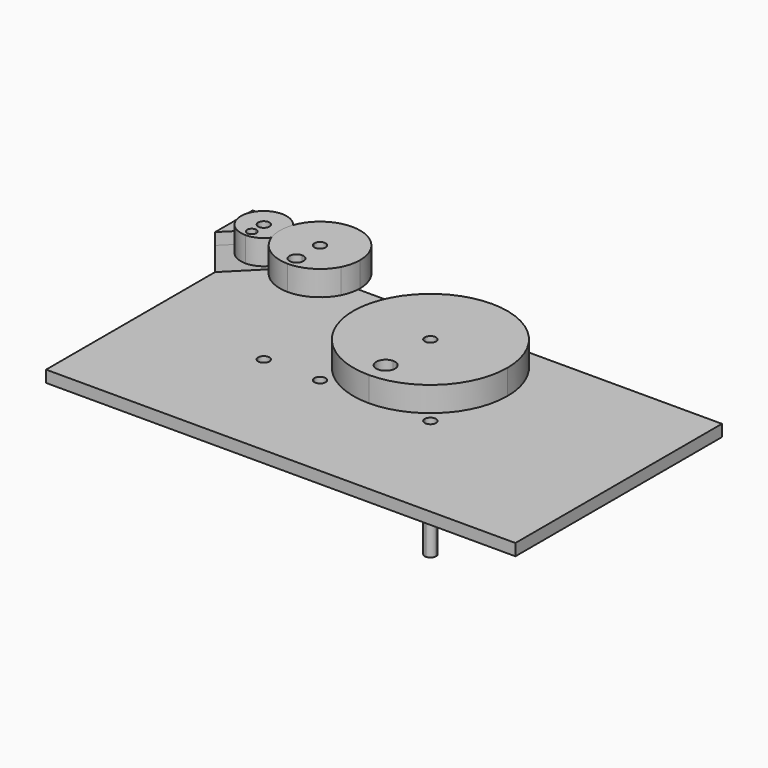
from build123d import *

# Parameters (mm, degrees)
F0_W     = 12.7
F0_H     = 6.35
F1_DEPTH = 3.175
F2_START = 25.4
F2_DEPTH = 6.731
F3_START = 25.4
F3_DEPTH = 6.731
F4_START = 12.7
F4_DEPTH = 6.731
F5_START = -6.35
F5_DEPTH = 25.4
F6_DEPTH = 6.35
F7_DEPTH = 3.175
F8_DEPTH = 6.35
F9_DEPTH = 3.175


# Not quite as in the source:
# - a feature names something its author has since deleted; it is built from what else it names


with BuildPart() as f1:
    # F0 (on Top) → F1 (new body)
    with BuildSketch(Plane.XY):
        Polygon((-53.6384286517, 34.5555226523), (-53.6384286517, 40.9055226523), (-66.3384286517, 28.2055226523), (-66.3384286517, -28.9444773477), (60.6615713483, -28.9444773477), (60.6615713483, 40.9055226523), (-40.9384286517, 40.9055226523), (-40.9384286517, 34.5555226523), align=None)
        with BuildLine():
            ThreePointArc((-33.3374786517, -2.7570773477), (-37.7198436388, -0.9418423348), (-39.5350786517, 3.4405226523))
            ThreePointArc((-39.5350786517, 3.4405226523), (-35.2680968666, 9.3297466308), (-28.3426948036, 7.1096342711))
            ThreePointArc((-28.3426948036, 7.1096342711), (-18.8492977605, 14.2746971722), (-8.4843562027, 8.4411133425))
            ThreePointArc((-8.4843562027, 8.4411133425), (14.2662795753, 24.1284571428), (32.5882213483, 3.4405226523))
            ThreePointArc((32.5882213483, 3.4405226523), (26.484121643, -11.2960776424), (11.7475213483, -17.4001773477))
            ThreePointArc((11.7475213483, -17.4001773477), (-1.1000263962, -12.9690871372), (-8.4843562027, -1.5600680379))
            ThreePointArc((-8.4843562027, -1.5600680379), (-12.5449573003, -5.8757972031), (-18.2667243218, -7.4170245234))
            ThreePointArc((-18.2667243218, -7.4170245234), (-24.4292066664, -5.3990050059), (-28.3426948036, -0.2285889665))
            ThreePointArc((-28.3426948036, -0.2285889665), (-30.5383216722, -2.0889407904), (-33.3374786517, -2.7570773477))
        make_face(mode=Mode.SUBTRACT)
        with BuildLine():
            ThreePointArc((32.5882213483, 3.4405226523), (14.2662795753, 24.1284571428), (-8.4843562027, 8.4411133425))
            ThreePointArc((-8.4843562027, 8.4411133425), (-7.5737811011, 6.0141510479), (-7.2643786517, 3.4405226523))
            Line((-7.2643786517, 3.4405226523), (-3.4734286517, 3.4405226523))
            Line((-3.4734286517, 3.4405226523), (10.2235213483, 3.4405226523))
            ThreePointArc((10.2235213483, 3.4405226523), (11.7475213483, 4.9645226523), (13.2715213483, 3.4405226523))
            Line((13.2715213483, 3.4405226523), (32.5882213483, 3.4405226523))
        make_face()
        with BuildLine():
            ThreePointArc((11.7475213483, -17.4001773477), (26.484121643, -11.2960776424), (32.5882213483, 3.4405226523))
            Line((32.5882213483, 3.4405226523), (13.2715213483, 3.4405226523))
            ThreePointArc((13.2715213483, 3.4405226523), (12.8251520828, 2.3628919178), (11.7475213483, 1.9165226523))
            Line((11.7475213483, 1.9165226523), (11.7475213483, -9.1447418249))
            ThreePointArc((11.7475213483, -9.1447418249), (13.5435725725, -9.8886906007), (14.2875213483, -11.6847418249))
            ThreePointArc((14.2875213483, -11.6847418249), (13.5435725725, -13.4807930491), (11.7475213483, -14.2247418249))
            Line((11.7475213483, -14.2247418249), (11.7475213483, -17.4001773477))
        make_face()
        with BuildLine():
            Line((-3.4734286517, 3.4405226523), (-7.2643786517, 3.4405226523))
            ThreePointArc((-7.2643786517, 3.4405226523), (-7.5737811011, 0.8668942566), (-8.4843562027, -1.5600680379))
            ThreePointArc((-8.4843562027, -1.5600680379), (-1.1000263962, -12.9690871372), (11.7475213483, -17.4001773477))
            Line((11.7475213483, -17.4001773477), (11.7475213483, -14.2247418249))
            ThreePointArc((11.7475213483, -14.2247418249), (9.2075213483, -11.6847418249), (11.7475213483, -9.1447418249))
            Line((11.7475213483, -9.1447418249), (11.7475213483, 1.9165226523))
            ThreePointArc((11.7475213483, 1.9165226523), (10.6698906138, 2.3628919178), (10.2235213483, 3.4405226523))
            Line((10.2235213483, 3.4405226523), (-3.4734286517, 3.4405226523))
        make_face()
        with BuildLine():
            ThreePointArc((-28.3426948036, 7.1096342711), (-27.4482546732, 5.3711408672), (-27.1398786517, 3.4405226523))
            Line((-27.1398786517, 3.4405226523), (-19.6468786517, 3.4405226523))
            ThreePointArc((-19.6468786517, 3.4405226523), (-18.1228786517, 4.9645226523), (-16.5988786517, 3.4405226523))
            Line((-16.5988786517, 3.4405226523), (-9.0931786517, 3.4405226523))
            ThreePointArc((-9.0931786517, 3.4405226523), (-8.9404131422, 5.9592808793), (-8.4843562027, 8.4411133425))
            ThreePointArc((-8.4843562027, 8.4411133425), (-18.8492977605, 14.2746971722), (-28.3426948036, 7.1096342711))
        make_face()
        Polygon((-53.6384286517, 40.9055226523), (-66.3384286517, 40.9055226523), (-66.3384286517, 28.2055226523), align=None)
        with Locations((-47.2884286517, 37.7305226523)):
            Rectangle(F0_W, F0_H)
        with BuildLine():
            Line((-19.6468786517, 3.4405226523), (-27.1398786517, 3.4405226523))
            ThreePointArc((-27.1398786517, 3.4405226523), (-27.4482546732, 1.5099044374), (-28.3426948036, -0.2285889665))
            ThreePointArc((-28.3426948036, -0.2285889665), (-24.4292066664, -5.3990050059), (-18.2667243218, -7.4170245234))
            Line((-18.2667243218, -7.4170245234), (-18.2516454134, -6.2788605557))
            ThreePointArc((-18.2516454134, -6.2788605557), (-20.1312421688, -4.3487916354), (-18.2011732485, -2.46919488))
            Line((-18.2011732485, -2.46919488), (-18.1430675177, 1.916656382))
            ThreePointArc((-18.1430675177, 1.916656382), (-19.2076237443, 2.3700535569), (-19.6468786517, 3.4405226523))
        make_face()
        with BuildLine():
            Line((-18.2516454134, -6.2788605557), (-18.2667243218, -7.4170245234))
            ThreePointArc((-18.2667243218, -7.4170245234), (-12.5449573003, -5.8757972031), (-8.4843562027, -1.5600680379))
            ThreePointArc((-8.4843562027, -1.5600680379), (-8.9404131422, 0.9217644253), (-9.0931786517, 3.4405226523))
            Line((-9.0931786517, 3.4405226523), (-16.5988786517, 3.4405226523))
            ThreePointArc((-16.5988786517, 3.4405226523), (-17.0524095563, 2.3557775597), (-18.1430675177, 1.916656382))
            Line((-18.1430675177, 1.916656382), (-18.2011732485, -2.46919488))
            ThreePointArc((-18.2011732485, -2.46919488), (-16.8704779652, -3.0359413487), (-16.321409331, -4.3740277179))
            ThreePointArc((-16.321409331, -4.3740277179), (-16.8883229618, -5.7299590836), (-18.2516454134, -6.2788605557))
        make_face()
        with BuildLine():
            ThreePointArc((-34.8614786517, 3.4405226523), (-33.3374786517, 4.9645226523), (-31.8134786517, 3.4405226523))
            Line((-31.8134786517, 3.4405226523), (-28.9813786517, 3.4405226523))
            ThreePointArc((-28.9813786517, 3.4405226523), (-28.8205161464, 5.3026650427), (-28.3426948036, 7.1096342711))
            ThreePointArc((-28.3426948036, 7.1096342711), (-35.2680968666, 9.3297466308), (-39.5350786517, 3.4405226523))
            Line((-39.5350786517, 3.4405226523), (-34.8614786517, 3.4405226523))
        make_face()
        with BuildLine():
            Line((-33.3374786517, 0.6427138499), (-33.3374786517, 1.9165226523))
            ThreePointArc((-33.3374786517, 1.9165226523), (-34.4151093862, 2.3628919178), (-34.8614786517, 3.4405226523))
            Line((-34.8614786517, 3.4405226523), (-39.5350786517, 3.4405226523))
            ThreePointArc((-39.5350786517, 3.4405226523), (-37.7198436388, -0.9418423348), (-33.3374786517, -2.7570773477))
            Line((-33.3374786517, -2.7570773477), (-33.3374786517, -1.8972861501))
            ThreePointArc((-33.3374786517, -1.8972861501), (-34.6074786517, -0.6272861501), (-33.3374786517, 0.6427138499))
        make_face()
        with BuildLine():
            Line((-28.9813786517, 3.4405226523), (-31.8134786517, 3.4405226523))
            ThreePointArc((-31.8134786517, 3.4405226523), (-32.2598479172, 2.3628919178), (-33.3374786517, 1.9165226523))
            Line((-33.3374786517, 1.9165226523), (-33.3374786517, 0.6427138499))
            ThreePointArc((-33.3374786517, 0.6427138499), (-32.4394530396, 0.270739462), (-32.0674786517, -0.6272861501))
            ThreePointArc((-32.0674786517, -0.6272861501), (-32.4394530396, -1.5253117622), (-33.3374786517, -1.8972861501))
            Line((-33.3374786517, -1.8972861501), (-33.3374786517, -2.7570773477))
            ThreePointArc((-33.3374786517, -2.7570773477), (-30.5383216722, -2.0889407904), (-28.3426948036, -0.2285889665))
            ThreePointArc((-28.3426948036, -0.2285889665), (-28.8205161464, 1.5783802619), (-28.9813786517, 3.4405226523))
        make_face()
        with BuildLine():
            Line((11.7475213483, -9.1447418249), (11.7475213483, -14.2247418249))
            ThreePointArc((11.7475213483, -14.2247418249), (13.5435725725, -13.4807930491), (14.2875213483, -11.6847418249))
            ThreePointArc((14.2875213483, -11.6847418249), (13.5435725725, -9.8886906007), (11.7475213483, -9.1447418249))
        make_face()
        with BuildLine():
            ThreePointArc((11.7475213483, -9.1447418249), (9.2075213483, -11.6847418249), (11.7475213483, -14.2247418249))
            Line((11.7475213483, -14.2247418249), (11.7475213483, -9.1447418249))
        make_face()
        with BuildLine():
            Line((-7.2643786517, 3.4405226523), (-9.0931786517, 3.4405226523))
            ThreePointArc((-9.0931786517, 3.4405226523), (-8.9404131422, 0.9217644253), (-8.4843562027, -1.5600680379))
            ThreePointArc((-8.4843562027, -1.5600680379), (-7.5737811011, 0.8668942566), (-7.2643786517, 3.4405226523))
        make_face()
        with BuildLine():
            ThreePointArc((-7.2643786517, 3.4405226523), (-7.5737811011, 6.0141510479), (-8.4843562027, 8.4411133425))
            ThreePointArc((-8.4843562027, 8.4411133425), (-8.9404131422, 5.9592808793), (-9.0931786517, 3.4405226523))
            Line((-9.0931786517, 3.4405226523), (-7.2643786517, 3.4405226523))
        make_face()
        with BuildLine():
            Line((-18.2011732485, -2.46919488), (-18.2516454134, -6.2788605557))
            ThreePointArc((-18.2516454134, -6.2788605557), (-16.8883229618, -5.7299590836), (-16.321409331, -4.3740277179))
            ThreePointArc((-16.321409331, -4.3740277179), (-16.8704779652, -3.0359413487), (-18.2011732485, -2.46919488))
        make_face()
        with BuildLine():
            ThreePointArc((-18.2011732485, -2.46919488), (-20.1312421688, -4.3487916354), (-18.2516454134, -6.2788605557))
            Line((-18.2516454134, -6.2788605557), (-18.2011732485, -2.46919488))
        make_face()
        with BuildLine():
            Line((-27.1398786517, 3.4405226523), (-28.9813786517, 3.4405226523))
            ThreePointArc((-28.9813786517, 3.4405226523), (-28.8205161464, 1.5783802619), (-28.3426948036, -0.2285889665))
            ThreePointArc((-28.3426948036, -0.2285889665), (-27.4482546732, 1.5099044374), (-27.1398786517, 3.4405226523))
        make_face()
        with BuildLine():
            ThreePointArc((-28.3426948036, 7.1096342711), (-28.8205161464, 5.3026650427), (-28.9813786517, 3.4405226523))
            Line((-28.9813786517, 3.4405226523), (-27.1398786517, 3.4405226523))
            ThreePointArc((-27.1398786517, 3.4405226523), (-27.4482546732, 5.3711408672), (-28.3426948036, 7.1096342711))
        make_face()
        with BuildLine():
            Line((-33.3374786517, -1.8972861501), (-33.3374786517, 0.6427138499))
            ThreePointArc((-33.3374786517, 0.6427138499), (-34.6074786517, -0.6272861501), (-33.3374786517, -1.8972861501))
        make_face()
        with BuildLine():
            ThreePointArc((-32.0674786517, -0.6272861501), (-32.4394530396, 0.270739462), (-33.3374786517, 0.6427138499))
            Line((-33.3374786517, 0.6427138499), (-33.3374786517, -1.8972861501))
            ThreePointArc((-33.3374786517, -1.8972861501), (-32.4394530396, -1.5253117622), (-32.0674786517, -0.6272861501))
        make_face()
    extrude(amount=-F1_DEPTH)


with BuildPart() as f2:
    # F0 (on Top) → F2 (new body)
    with BuildSketch(Plane.XY.offset(F2_START)):
        with BuildLine():
            ThreePointArc((-34.8614786517, 3.4405226523), (-33.3374786517, 4.9645226523), (-31.8134786517, 3.4405226523))
            Line((-31.8134786517, 3.4405226523), (-28.9813786517, 3.4405226523))
            ThreePointArc((-28.9813786517, 3.4405226523), (-28.8205161464, 5.3026650427), (-28.3426948036, 7.1096342711))
            ThreePointArc((-28.3426948036, 7.1096342711), (-35.2680968666, 9.3297466308), (-39.5350786517, 3.4405226523))
            Line((-39.5350786517, 3.4405226523), (-34.8614786517, 3.4405226523))
        make_face()
        with BuildLine():
            Line((-33.3374786517, 0.6427138499), (-33.3374786517, 1.9165226523))
            ThreePointArc((-33.3374786517, 1.9165226523), (-34.4151093862, 2.3628919178), (-34.8614786517, 3.4405226523))
            Line((-34.8614786517, 3.4405226523), (-39.5350786517, 3.4405226523))
            ThreePointArc((-39.5350786517, 3.4405226523), (-37.7198436388, -0.9418423348), (-33.3374786517, -2.7570773477))
            Line((-33.3374786517, -2.7570773477), (-33.3374786517, -1.8972861501))
            ThreePointArc((-33.3374786517, -1.8972861501), (-34.6074786517, -0.6272861501), (-33.3374786517, 0.6427138499))
        make_face()
        with BuildLine():
            Line((-28.9813786517, 3.4405226523), (-31.8134786517, 3.4405226523))
            ThreePointArc((-31.8134786517, 3.4405226523), (-32.2598479172, 2.3628919178), (-33.3374786517, 1.9165226523))
            Line((-33.3374786517, 1.9165226523), (-33.3374786517, 0.6427138499))
            ThreePointArc((-33.3374786517, 0.6427138499), (-32.4394530396, 0.270739462), (-32.0674786517, -0.6272861501))
            ThreePointArc((-32.0674786517, -0.6272861501), (-32.4394530396, -1.5253117622), (-33.3374786517, -1.8972861501))
            Line((-33.3374786517, -1.8972861501), (-33.3374786517, -2.7570773477))
            ThreePointArc((-33.3374786517, -2.7570773477), (-30.5383216722, -2.0889407904), (-28.3426948036, -0.2285889665))
            ThreePointArc((-28.3426948036, -0.2285889665), (-28.8205161464, 1.5783802619), (-28.9813786517, 3.4405226523))
        make_face()
        with BuildLine():
            Line((-27.1398786517, 3.4405226523), (-28.9813786517, 3.4405226523))
            ThreePointArc((-28.9813786517, 3.4405226523), (-28.8205161464, 1.5783802619), (-28.3426948036, -0.2285889665))
            ThreePointArc((-28.3426948036, -0.2285889665), (-27.4482546732, 1.5099044374), (-27.1398786517, 3.4405226523))
        make_face()
        with BuildLine():
            ThreePointArc((-28.3426948036, 7.1096342711), (-28.8205161464, 5.3026650427), (-28.9813786517, 3.4405226523))
            Line((-28.9813786517, 3.4405226523), (-27.1398786517, 3.4405226523))
            ThreePointArc((-27.1398786517, 3.4405226523), (-27.4482546732, 5.3711408672), (-28.3426948036, 7.1096342711))
        make_face()
    extrude(amount=F2_DEPTH)


with BuildPart() as f3:
    # F0 (on Top) → F3 (new body)
    with BuildSketch(Plane.XY.offset(F3_START)):
        with BuildLine():
            ThreePointArc((-28.3426948036, 7.1096342711), (-27.4482546732, 5.3711408672), (-27.1398786517, 3.4405226523))
            Line((-27.1398786517, 3.4405226523), (-19.6468786517, 3.4405226523))
            ThreePointArc((-19.6468786517, 3.4405226523), (-18.1228786517, 4.9645226523), (-16.5988786517, 3.4405226523))
            Line((-16.5988786517, 3.4405226523), (-9.0931786517, 3.4405226523))
            ThreePointArc((-9.0931786517, 3.4405226523), (-8.9404131422, 5.9592808793), (-8.4843562027, 8.4411133425))
            ThreePointArc((-8.4843562027, 8.4411133425), (-18.8492977605, 14.2746971722), (-28.3426948036, 7.1096342711))
        make_face()
        with BuildLine():
            Line((-19.6468786517, 3.4405226523), (-27.1398786517, 3.4405226523))
            ThreePointArc((-27.1398786517, 3.4405226523), (-27.4482546732, 1.5099044374), (-28.3426948036, -0.2285889665))
            ThreePointArc((-28.3426948036, -0.2285889665), (-24.4292066664, -5.3990050059), (-18.2667243218, -7.4170245234))
            Line((-18.2667243218, -7.4170245234), (-18.2516454134, -6.2788605557))
            ThreePointArc((-18.2516454134, -6.2788605557), (-20.1312421688, -4.3487916354), (-18.2011732485, -2.46919488))
            Line((-18.2011732485, -2.46919488), (-18.1430675177, 1.916656382))
            ThreePointArc((-18.1430675177, 1.916656382), (-19.2076237443, 2.3700535569), (-19.6468786517, 3.4405226523))
        make_face()
        with BuildLine():
            Line((-18.2516454134, -6.2788605557), (-18.2667243218, -7.4170245234))
            ThreePointArc((-18.2667243218, -7.4170245234), (-12.5449573003, -5.8757972031), (-8.4843562027, -1.5600680379))
            ThreePointArc((-8.4843562027, -1.5600680379), (-8.9404131422, 0.9217644253), (-9.0931786517, 3.4405226523))
            Line((-9.0931786517, 3.4405226523), (-16.5988786517, 3.4405226523))
            ThreePointArc((-16.5988786517, 3.4405226523), (-17.0524095563, 2.3557775597), (-18.1430675177, 1.916656382))
            Line((-18.1430675177, 1.916656382), (-18.2011732485, -2.46919488))
            ThreePointArc((-18.2011732485, -2.46919488), (-16.8704779652, -3.0359413487), (-16.321409331, -4.3740277179))
            ThreePointArc((-16.321409331, -4.3740277179), (-16.8883229618, -5.7299590836), (-18.2516454134, -6.2788605557))
        make_face()
        with BuildLine():
            ThreePointArc((-28.3426948036, 7.1096342711), (-28.8205161464, 5.3026650427), (-28.9813786517, 3.4405226523))
            Line((-28.9813786517, 3.4405226523), (-27.1398786517, 3.4405226523))
            ThreePointArc((-27.1398786517, 3.4405226523), (-27.4482546732, 5.3711408672), (-28.3426948036, 7.1096342711))
        make_face()
        with BuildLine():
            Line((-27.1398786517, 3.4405226523), (-28.9813786517, 3.4405226523))
            ThreePointArc((-28.9813786517, 3.4405226523), (-28.8205161464, 1.5783802619), (-28.3426948036, -0.2285889665))
            ThreePointArc((-28.3426948036, -0.2285889665), (-27.4482546732, 1.5099044374), (-27.1398786517, 3.4405226523))
        make_face()
        with BuildLine():
            ThreePointArc((-7.2643786517, 3.4405226523), (-7.5737811011, 6.0141510479), (-8.4843562027, 8.4411133425))
            ThreePointArc((-8.4843562027, 8.4411133425), (-8.9404131422, 5.9592808793), (-9.0931786517, 3.4405226523))
            Line((-9.0931786517, 3.4405226523), (-7.2643786517, 3.4405226523))
        make_face()
        with BuildLine():
            Line((-7.2643786517, 3.4405226523), (-9.0931786517, 3.4405226523))
            ThreePointArc((-9.0931786517, 3.4405226523), (-8.9404131422, 0.9217644253), (-8.4843562027, -1.5600680379))
            ThreePointArc((-8.4843562027, -1.5600680379), (-7.5737811011, 0.8668942566), (-7.2643786517, 3.4405226523))
        make_face()
    extrude(amount=F3_DEPTH)


with BuildPart() as f4:
    # F0 (on Top) → F4 (new body)
    with BuildSketch(Plane.XY.offset(F4_START)):
        with BuildLine():
            ThreePointArc((-7.2643786517, 3.4405226523), (-7.5737811011, 6.0141510479), (-8.4843562027, 8.4411133425))
            ThreePointArc((-8.4843562027, 8.4411133425), (-8.9404131422, 5.9592808793), (-9.0931786517, 3.4405226523))
            Line((-9.0931786517, 3.4405226523), (-7.2643786517, 3.4405226523))
        make_face()
        with BuildLine():
            ThreePointArc((32.5882213483, 3.4405226523), (14.2662795753, 24.1284571428), (-8.4843562027, 8.4411133425))
            ThreePointArc((-8.4843562027, 8.4411133425), (-7.5737811011, 6.0141510479), (-7.2643786517, 3.4405226523))
            Line((-7.2643786517, 3.4405226523), (-3.4734286517, 3.4405226523))
            Line((-3.4734286517, 3.4405226523), (10.2235213483, 3.4405226523))
            ThreePointArc((10.2235213483, 3.4405226523), (11.7475213483, 4.9645226523), (13.2715213483, 3.4405226523))
            Line((13.2715213483, 3.4405226523), (32.5882213483, 3.4405226523))
        make_face()
        with BuildLine():
            ThreePointArc((11.7475213483, -17.4001773477), (26.484121643, -11.2960776424), (32.5882213483, 3.4405226523))
            Line((32.5882213483, 3.4405226523), (13.2715213483, 3.4405226523))
            ThreePointArc((13.2715213483, 3.4405226523), (12.8251520828, 2.3628919178), (11.7475213483, 1.9165226523))
            Line((11.7475213483, 1.9165226523), (11.7475213483, -9.1447418249))
            ThreePointArc((11.7475213483, -9.1447418249), (13.5435725725, -9.8886906007), (14.2875213483, -11.6847418249))
            ThreePointArc((14.2875213483, -11.6847418249), (13.5435725725, -13.4807930491), (11.7475213483, -14.2247418249))
            Line((11.7475213483, -14.2247418249), (11.7475213483, -17.4001773477))
        make_face()
        with BuildLine():
            Line((-7.2643786517, 3.4405226523), (-9.0931786517, 3.4405226523))
            ThreePointArc((-9.0931786517, 3.4405226523), (-8.9404131422, 0.9217644253), (-8.4843562027, -1.5600680379))
            ThreePointArc((-8.4843562027, -1.5600680379), (-7.5737811011, 0.8668942566), (-7.2643786517, 3.4405226523))
        make_face()
        with BuildLine():
            Line((-3.4734286517, 3.4405226523), (-7.2643786517, 3.4405226523))
            ThreePointArc((-7.2643786517, 3.4405226523), (-7.5737811011, 0.8668942566), (-8.4843562027, -1.5600680379))
            ThreePointArc((-8.4843562027, -1.5600680379), (-1.1000263962, -12.9690871372), (11.7475213483, -17.4001773477))
            Line((11.7475213483, -17.4001773477), (11.7475213483, -14.2247418249))
            ThreePointArc((11.7475213483, -14.2247418249), (9.2075213483, -11.6847418249), (11.7475213483, -9.1447418249))
            Line((11.7475213483, -9.1447418249), (11.7475213483, 1.9165226523))
            ThreePointArc((11.7475213483, 1.9165226523), (10.6698906138, 2.3628919178), (10.2235213483, 3.4405226523))
            Line((10.2235213483, 3.4405226523), (-3.4734286517, 3.4405226523))
        make_face()
    extrude(amount=F4_DEPTH)


with BuildPart() as f5:
    # F0 (on Top) → F5 (new body)
    with BuildSketch(Plane.XY.offset(F5_START)):
        with BuildLine():
            Line((11.7475213483, 3.4405226523), (13.2715213483, 3.4405226523))
            ThreePointArc((13.2715213483, 3.4405226523), (11.7475213483, 4.9645226523), (10.2235213483, 3.4405226523))
            Line((10.2235213483, 3.4405226523), (11.7475213483, 3.4405226523))
        make_face()
        with BuildLine():
            Line((11.7475213483, 3.4405226523), (10.2235213483, 3.4405226523))
            ThreePointArc((10.2235213483, 3.4405226523), (10.6698906138, 2.3628919178), (11.7475213483, 1.9165226523))
            Line((11.7475213483, 1.9165226523), (11.7475213483, 3.4405226523))
        make_face()
        with BuildLine():
            ThreePointArc((11.7475213483, 1.9165226523), (12.8251520828, 2.3628919178), (13.2715213483, 3.4405226523))
            Line((13.2715213483, 3.4405226523), (11.7475213483, 3.4405226523))
            Line((11.7475213483, 3.4405226523), (11.7475213483, 1.9165226523))
        make_face()
    extrude(amount=-F5_DEPTH)


with BuildPart() as f6:
    # F0 (on Top) → F6 (new body)
    with BuildSketch(Plane.XY):
        Polygon((-53.6384286517, 40.9055226523), (-66.3384286517, 40.9055226523), (-66.3384286517, 28.2055226523), align=None)
    extrude(amount=F6_DEPTH)


with BuildPart() as f7:
    # F7 (new): a face of the model
    f7_faces = [f6.part.faces().sort_by_distance(p)[0] for p in [
        (-62.1050953184, 36.672189319, 6.35),
    ]]
    extrude(f7_faces, amount=F7_DEPTH)


with BuildPart() as f8:
    # F0 (on Top) → F8 (new body)
    with BuildSketch(Plane.XY):
        with Locations((-47.2884286517, 37.7305226523)):
            Rectangle(F0_W, F0_H)
    extrude(amount=F8_DEPTH)


with BuildPart() as f9:
    # F9 (new): a face of the model
    f9_faces = [f8.part.faces().sort_by_distance(p)[0] for p in [
        (-47.2884286517, 37.7305226523, 6.35),
    ]]
    extrude(f9_faces, amount=F9_DEPTH)


solid = Compound([f1.part, f2.part, f3.part, f4.part, f5.part, f6.part, f7.part, f8.part, f9.part])
